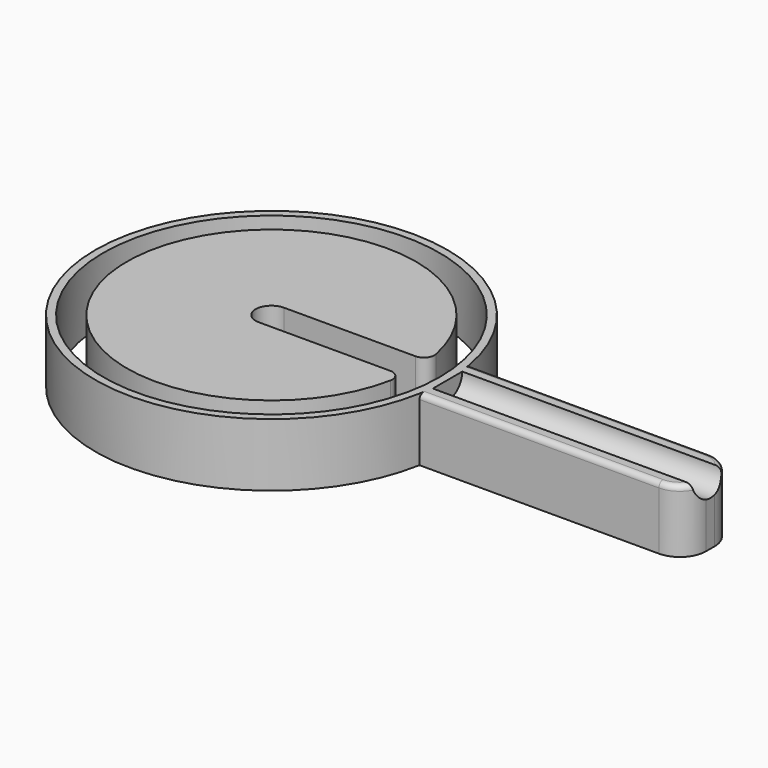
from build123d import *

# Parameters (mm, degrees)
F1_DEPTH     = 12
F2_R         = 2
F3_R         = 32
F4_DEPTH     = 12
F6_DEPTH     = 50
F7_T1_DEPTH  = 37
F8_T4_DEPTH  = 48.0416930046
F8_S5_R      = 33.5
F8_T6_DEPTH  = 26
F8_T10_DEPTH = 48.0416930046
F8_S11_R     = 33.5
F8_T12_DEPTH = 26
F8_T14_ANGLE = 88.6530036621
F8_T16_ANGLE = 88.6530036621


# Not quite as in the source:
# - a fillet or chamfer that OpenCascade refuses, or shapes differently, is made with other operations: its cross-section is extruded or revolved along the edge and cut away or added


with BuildPart() as f1:
    # F0 (on Top) → F1 (new body)
    with BuildSketch(Plane.XY):
        with BuildLine():
            Line((0, 3), (27.3358738657, 3))
            ThreePointArc((27.3358738657, 3), (-27.5, 0), (27.3358738657, -3))
            Line((27.3358738657, -3), (0, -3))
            ThreePointArc((0, -3), (-3, 0), (0, 3))
        make_face()
    extrude(amount=F1_DEPTH)

    # F2
    f2_edges = [f1.edges().sort_by_distance(p)[0] for p in [
        (27.335874, 3, 6),
        (27.335874, -3, 6),
    ]]
    fillet(f2_edges, radius=F2_R)


with BuildPart() as f4:
    # F3 (on Top) → F4 (new body)
    with BuildSketch(Plane.XY):
        with BuildLine():
            Line((83.5, 6), (32.9583069954, 6))
            ThreePointArc((32.9583069954, 6), (-33.5, 0), (32.9583069954, -6))
            Line((32.9583069954, -6), (83.5, -6))
            Line((83.5, -6), (83.5, 6))
        make_face()
        Circle(F3_R, mode=Mode.SUBTRACT)
    extrude(amount=F4_DEPTH)

    # F5 (on face) → F6 (cut)
    with BuildSketch(Plane.YZ.offset(83.5)):
        with BuildLine():
            ThreePointArc((-3.5, 12), (0, 8.5), (3.5, 12))
            Line((3.5, 12), (-3.5, 12))
        make_face()
    extrude(amount=-F6_DEPTH, mode=Mode.SUBTRACT)

    # F7: fillet of radius 5 on 2 edges, made by hand

    # F7_s2 → F7_t1 (cut)
    with BuildSketch(Plane.XY.offset(-12.5)):
        with BuildLine():
            ThreePointArc((78.5, -6), (82.0355339059, -4.5355339059), (83.5, -1))
            Line((83.5, -1), (83.5, -6))
            Line((83.5, -6), (78.5, -6))
        make_face()
        with BuildLine():
            ThreePointArc((83.5, 1), (82.0355339059, 4.5355339059), (78.5, 6))
            Line((78.5, 6), (83.5, 6))
            Line((83.5, 6), (83.5, 1))
        make_face()
    extrude(amount=F7_T1_DEPTH, mode=Mode.SUBTRACT)

    # F8: fillet of radius 1 on 2 edges, made by hand


with BuildPart() as f8_tool2:
    # F8_s3 → F8_t4 (new body)
    with BuildSketch(Plane.YZ.offset(30.4583069954)):
        with BuildLine():
            ThreePointArc((-6, 11), (-5.7071067812, 11.7071067812), (-5, 12))
            Line((-5, 12), (-6, 12))
            Line((-6, 12), (-6, 11))
        make_face()
    extrude(amount=F8_T4_DEPTH)

    # F8_s5 → F8_t6 (cut, symmetric)
    with BuildSketch(Plane.XY.offset(11.5)):
        Circle(F8_S5_R)
    extrude(amount=F8_T6_DEPTH, both=True, mode=Mode.SUBTRACT)


with BuildPart() as f4_1:
    add(f4.part)

    # F8_t1: cut F8_tool2
    add(f8_tool2.part, mode=Mode.SUBTRACT)


with BuildPart() as f8_tool8:
    # F8_s9 → F8_t10 (new body)
    with BuildSketch(Plane.YZ.offset(78.5)):
        with BuildLine():
            ThreePointArc((5, 12), (5.7071067812, 11.7071067812), (6, 11))
            Line((6, 11), (6, 12))
            Line((6, 12), (5, 12))
        make_face()
    extrude(amount=-F8_T10_DEPTH)

    # F8_s11 → F8_t12 (cut, symmetric)
    with BuildSketch(Plane.XY.offset(11.5)):
        Circle(F8_S11_R)
    extrude(amount=F8_T12_DEPTH, both=True, mode=Mode.SUBTRACT)


with BuildPart() as f4_2:
    add(f4_1.part)

    # F8_t7: cut F8_tool8
    add(f8_tool8.part, mode=Mode.SUBTRACT)

    # F8_s13 → F8_t14 (revolve, cut)
    with BuildSketch(Plane.YZ.offset(78.4999999999)):
        with BuildLine():
            ThreePointArc((5, 12), (5.7071067812, 11.7071067812), (6, 11))
            Line((6, 11), (6, 12))
            Line((6, 12), (5, 12))
        make_face()
    revolve(axis=Axis((78.4999999999, 0.9999999999, 12), (0, 0, -1)), revolution_arc=F8_T14_ANGLE, mode=Mode.SUBTRACT)

    # F8_s15 → F8_t16 (revolve, cut)
    with BuildSketch(Plane(origin=(0.0198779079, 0.845370075, 0), x_dir=(0, 0, 1), z_dir=(0.0235073555, 0.9997236639, 0))):
        with BuildLine():
            ThreePointArc((11, 83.5018149746), (11.7071067812, 83.2089217558), (12, 82.5018149746))
            Line((12, 82.5018149746), (12, 83.5018149746))
            Line((12, 83.5018149746), (11, 83.5018149746))
        make_face()
    revolve(axis=Axis((78.4999999999, -0.9999999999, 12), (0, 0, -1)), revolution_arc=F8_T16_ANGLE, mode=Mode.SUBTRACT)


solid = Compound([f1.part, f4_2.part])
